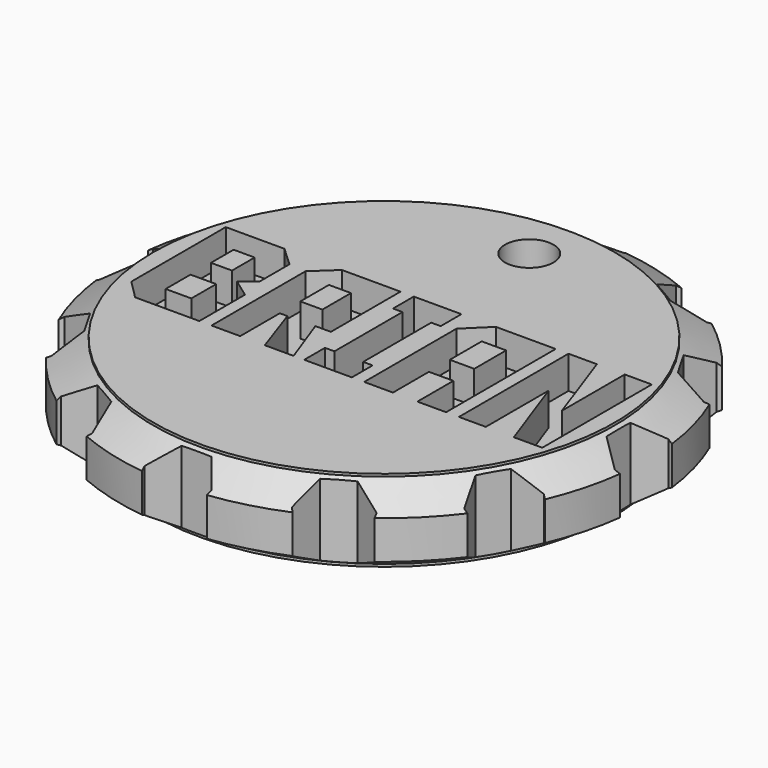
from build123d import *

# Parameters (mm, degrees)
F4_DEPTH        = 25.4
F4_COPIES_COUNT = 12
F5_R            = 1.4771792176
F6_DEPTH        = 25.4
F7_W            = 1.5664739324
F7_H            = 1.8959537424
F7_W_2          = 1.2832369833
F7_H_2          = 1.7283237234
F7_W_3          = 1.3468208245
F7_H_3          = 2.1791908396
F7_W_4          = 1.4913294871
F7_H_4          = 2.4335260562
F8_DEPTH        = 4


# Not quite as in the source:
# - a pattern or mirror of a feature is missing from the dataset's text; its kind, count and spacing are read off the source's solid


with BuildPart() as f1:
    # F0 (on Front) → F1 (revolve)
    with BuildSketch(Plane.XZ):
        Polygon((-14.078464359, 0), (0, 0), (0, 5), (-14.078464359, 5), (-14.078464359, 4.8446745319), (-14.078464359, 0.1553254681), align=None)
        Polygon((-16.1090120673, 1.327662734), (-14.078464359, 0.1553254681), (-14.078464359, 4.8446745319), (-16.1090120673, 3.672337266), align=None)
    revolve(axis=Axis((0, 0, 2.5), (0, 0, 1)))

    # F3 (on offset) → F4 (cut)
    with BuildSketch(Plane.XY.offset(7)):
        Polygon((-0.9072549192, 14.3041582778), (0.9072549192, 14.3041582778), (2.0385832989, 15.7227991948), (1.634816875, 17.4918154833), (0, 18.2791017967), (-1.634816875, 17.4918154833), (-2.0385832989, 15.7227991948), align=None)
    f4 = extrude(amount=-F4_DEPTH, mode=Mode.SUBTRACT)

    # F4_copies: F4 ×12 about axis
    f4_copies_axis = Axis((0, 0, 0), (0, 0, 1))
    for i in range(1, F4_COPIES_COUNT):
        add(f4.rotate(f4_copies_axis, i * 360 / F4_COPIES_COUNT), mode=Mode.SUBTRACT)

    # F5 (on offset) → F6 (cut)
    with BuildSketch(Plane.XY.offset(7)):
        with Locations((0, 11.0796838999)):
            Circle(F5_R)
    extrude(amount=-F6_DEPTH, mode=Mode.SUBTRACT)

    # F7 (on offset) → F8 (cut)
    with BuildSketch(Plane.XY.offset(7)):
        Polygon((-7.9248555319, -4.1791779859), (-7.9248555319, -0.6994093307), (-9.0520231003, 0.1156197041), (-8.2312138374, 0.7745791761), (-8.2312138374, 3.0751571738), (-9.416185019, 4.1792033859), (-13, 4.1792033859), (-13, -3.0231086849), (-11.843930699, -4.1791779859), align=None)
        with Locations((-10.465317954, -1.6473862019)):
            Rectangle(F7_W, F7_H, mode=Mode.SUBTRACT)
        with Locations((-10.6069364286, 1.7254462353)):
            Rectangle(F7_W_2, F7_H_2, mode=Mode.SUBTRACT)
        Polygon((-4.9710982903, -1.156056675), (-3.9306357714, -4.1791779859), (-2.1734104635, -4.1791779859), (-3.2832370516, -1.1329353186), (-2.3352601064, -1.1329353186), (-2.3352601064, 4.1792033859), (-5.9132948594, 4.1792033859), (-7.1849710904, 3.0000127285), (-7.1849710904, -4.1791779859), (-5.4335260106, -4.1791779859), (-5.4335260106, -1.156056675), align=None)
        with Locations((-4.7601155984, 1.5000126772)):
            Rectangle(F7_W_3, F7_H_3, mode=Mode.SUBTRACT)
        Polygon((1.3815029331, -4.1791779859), (1.3815029331, -2.5953630731), (0.8034681346, -2.5953630731), (0.8034681346, 2.5953884731), (1.3815029331, 2.5953884731), (1.3815029331, 4.1792033859), (-1.5260115957, 4.1792033859), (-1.5260115957, 2.5953884731), (-0.9479769452, 2.5953884731), (-0.9479769452, -2.5953630731), (-1.5260115957, -2.5953630731), (-1.5260115957, -4.1791779859), align=None)
        Polygon((2.1329479787, -4.1791779859), (3.8901734346, -4.1791779859), (3.8901734346, -1.433513248), (5.3815029217, -1.433513248), (5.3815029217, -4.1791779859), (7.1329480015, -4.1791779859), (7.1329480015, 4.1792033859), (3.4797688032, 4.1792033859), (2.1329479787, 2.8555040658), align=None)
        with Locations((4.6358381782, 1.3728450689)):
            Rectangle(F7_W_4, F7_H_4, mode=Mode.SUBTRACT)
        Polygon((11.34682087, 4.1792033859), (11.34682087, -0.6184843612), (9.6473988791, 4.1792033859), (7.9132947796, 4.1792033859), (7.9132947796, -4.1791779859), (9.5549133055, -4.1791779859), (9.5549133055, 0.6185097612), (11.2658959005, -4.1791779859), (13, -4.1791779859), (13, 4.1792033859), align=None)
    extrude(amount=-F8_DEPTH, mode=Mode.SUBTRACT)


solid = f1.part
